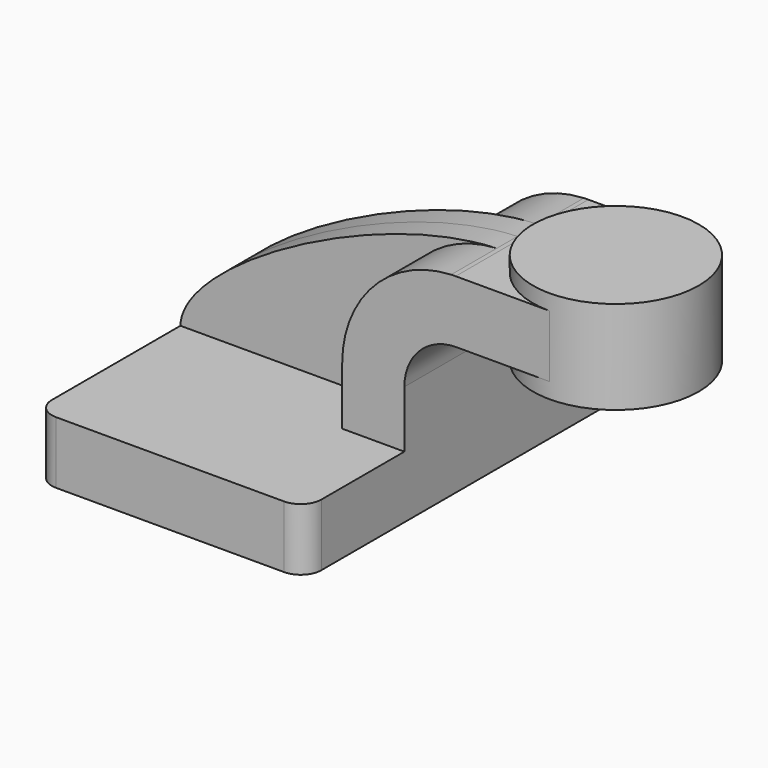
from build123d import *

# Parameters (mm, degrees)
F1_DEPTH = 63.5
F0_W     = 25.4
F0_H     = 19.05
F2_DEPTH = 25.4
F3_DEPTH = 7.9375
F5_R     = 6.35


# Not quite as in the source:
# - a feature names something its author has since deleted; it is built from what else it names


with BuildPart() as f1:
    # F0 (on Front) → F1 (new body, symmetric)
    with BuildSketch(Plane.XZ):
        Polygon((41.275, -9.525), (41.275, 9.525), (22.225, 9.525), (-41.275, 9.525), (-41.275, -9.525), align=None)
    extrude(amount=F1_DEPTH, both=True)

    # F0 (on Front) → F2 (join, symmetric)
    with BuildSketch(Plane.XZ):
        with BuildLine():
            Line((22.225, 9.525), (41.275, 9.525))
            Line((41.275, 9.525), (41.275, 27.0006215875))
            ThreePointArc((41.275, 27.0006215875), (45.9656588405, 38.2667716764), (57.2656945294, 42.8752))
            Line((57.2656945294, 42.8752), (60.325, 42.8752))
            Line((60.325, 42.8752), (60.325, 61.9252))
            Line((60.325, 61.9252), (56.9783966597, 61.9252))
            add(Edge.make_bspline(
                [(55.5906283852, 61.8907919104), (56.0567092962, 61.9071657032), (56.5193514661, 61.918664428), (56.9783966597, 61.9252)],
                knots=[109.9767617242, 109.9767617242, 109.9767617242, 109.9767617242, 111.3530911794, 111.3530911794, 111.3530911794, 111.3530911794], degree=3))
            ThreePointArc((55.5906283852, 61.8907919104), (31.9089948829, 51.1387094503), (22.225, 27.0006215875))
            Line((22.225, 27.0006215875), (22.225, 9.525))
        make_face()
        with Locations((73.025, 52.4002)):
            Rectangle(F0_W, F0_H)
    extrude(amount=F2_DEPTH, both=True)

    # F0 (on Front) → F3 (join, symmetric)
    with BuildSketch(Plane.XZ):
        with BuildLine():
            Line((-41.275, 9.525), (22.225, 9.525))
            Line((22.225, 9.525), (22.225, 27.0006215875))
            ThreePointArc((22.225, 27.0006215875), (31.9089948829, 51.1387094503), (55.5906283852, 61.8907919104))
            add(Edge.make_bspline(
                [(-41.275, 9.525), (-40.8507124628, 28.1470359497), (18.3480415197, 60.5824302397), (55.5906283852, 61.8907919104)],
                knots=[0, 0, 0, 0, 109.9767617242, 109.9767617242, 109.9767617242, 109.9767617242], degree=3))
        make_face()
    extrude(amount=F3_DEPTH, both=True)

    # F0 (on Front) → F4 (revolve)
    with BuildSketch(Plane.XZ):
        Polygon((85.725, 61.9252), (85.725, 42.8752), (85.725, 38.1), (111.125, 38.1), (111.125, 66.675), (85.725, 66.675), align=None)
    revolve(axis=Axis((85.725, 0, 52.3875), (0, 0, 1)))

    # F5
    f5_edges = [f1.edges().sort_by_distance(p)[0] for p in [
        (-41.275, -63.5, 0),
        (41.275, -63.5, 0),
        (41.275, 63.5, 0),
        (-41.275, 63.5, 0),
    ]]
    fillet(f5_edges, radius=F5_R)


solid = f1.part
